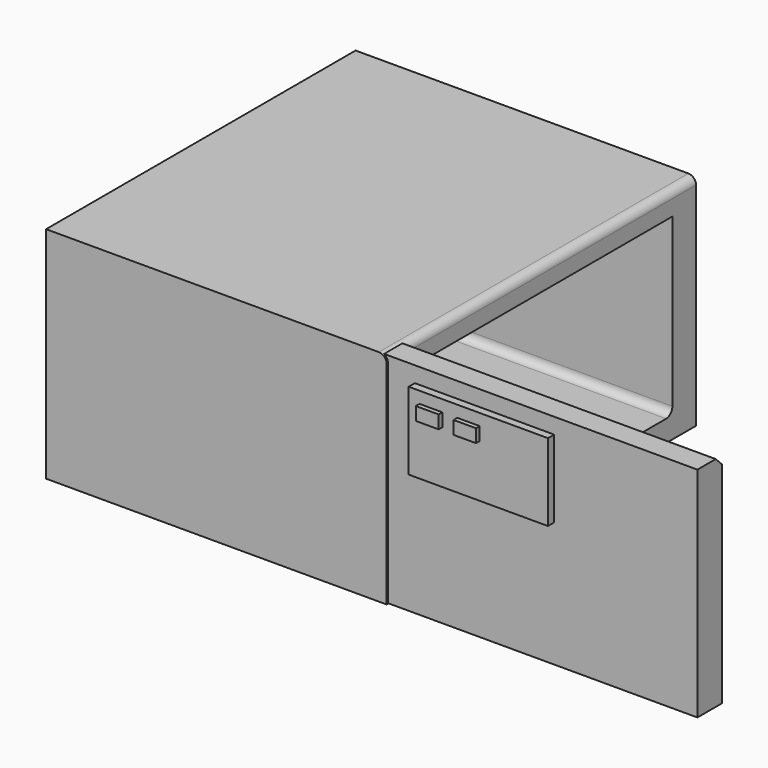
from build123d import *

# Parameters (mm, degrees)
F0_W         = 220
F0_H         = 141.9456327772
F1_DEPTH     = 250
F3_W         = 210.672037676
F3_H         = 112.9930540919
F4_DEPTH     = 206
F5_W         = 19.7831674727
F5_H         = 141
F6_DEPTH     = 200
F7_T4_DEPTH  = 275
F7_T10_DEPTH = 275
F7_T16_DEPTH = 275
F7_T23_DEPTH = 275
F7_T29_DEPTH = 275
F8_SIZE      = 5
F9_T1_DEPTH  = 218.5
F10_R        = 5
F11_R        = 5
F12_W        = 90
F12_H        = 50
F13_DEPTH    = 5
F14_W        = 14.7826219899
F14_H        = 8.5
F15_DEPTH    = 3
F16_W        = 14.5
F16_H        = 8.5
F17_DEPTH    = 3


# Not quite as in the source:
# - a fillet or chamfer that OpenCascade refuses, or shapes differently, is made with other operations: its cross-section is extruded or revolved along the edge and cut away or added


with BuildPart() as f1:
    # F0 (on Front) → F1 (new body)
    with BuildSketch(Plane.XZ):
        Rectangle(F0_W, F0_H)
    extrude(amount=F1_DEPTH)

    # F3 (on face) → F4 (cut)
    with BuildSketch(Plane.YZ.offset(110)):
        with Locations((-124.4797622785, -0.6201006472)):
            Rectangle(F3_W, F3_H)
    extrude(amount=-F4_DEPTH, mode=Mode.SUBTRACT)

    # F5 (on face) → F6 (join)
    with BuildSketch(Plane.YZ.offset(110)):
        with Locations((-239.0063405037, -0.1803636551)):
            Rectangle(F5_W, F5_H)
    extrude(amount=F6_DEPTH)

    # F7: fillet of radius 5 on 1 edges, made by hand


with BuildPart() as f7_tool2:
    # F7_s3 → F7_t4 (new body)
    with BuildSketch(Plane.XZ.offset(-12.5)):
        with BuildLine():
            ThreePointArc((105, 70.9728163886), (108.5355339059, 69.5083502945), (110, 65.9728163886))
            Line((110, 65.9728163886), (110, 70.9728163886))
            Line((110, 70.9728163886), (105, 70.9728163886))
        make_face()
    extrude(amount=F7_T4_DEPTH)

    split(bisect_by=Plane.XY.offset(70.3196363449), keep=Keep.TOP)

    split(bisect_by=Plane.XZ.offset(229.1147567674), keep=Keep.BOTTOM)


with BuildPart() as f1_1:
    add(f1.part)

    # F7_t1: cut F7_tool2
    add(f7_tool2.part, mode=Mode.SUBTRACT)


with BuildPart() as f7_tool8:
    # F7_s9 → F7_t10 (new body)
    with BuildSketch(Plane.XZ.offset(-12.5)):
        with BuildLine():
            ThreePointArc((105, 70.9728163886), (108.5355339059, 69.5083502945), (110, 65.9728163886))
            Line((110, 65.9728163886), (110, 70.9728163886))
            Line((110, 70.9728163886), (105, 70.9728163886))
        make_face()
    extrude(amount=F7_T10_DEPTH)

    split(bisect_by=Plane.XY.offset(70.3196363449), keep=Keep.BOTTOM)

    split(bisect_by=Plane.XZ.offset(229.1147567674), keep=Keep.BOTTOM)


with BuildPart() as f1_2:
    add(f1_1.part)

    # F7_t7: cut F7_tool8
    add(f7_tool8.part, mode=Mode.SUBTRACT)


with BuildPart() as f7_tool14:
    # F7_s15 → F7_t16 (new body)
    with BuildSketch(Plane.XZ.offset(-12.5)):
        with BuildLine():
            ThreePointArc((105, 70.9728163886), (108.5355339059, 69.5083502945), (110, 65.9728163886))
            Line((110, 65.9728163886), (110, 70.9728163886))
            Line((110, 70.9728163886), (105, 70.9728163886))
        make_face()
    extrude(amount=F7_T16_DEPTH)

    split(bisect_by=Plane.XZ.offset(248.89792424), keep=Keep.BOTTOM)

    split(bisect_by=Plane.XY.offset(70.3196363449), keep=Keep.TOP)

    split(bisect_by=Plane.XZ.offset(229.1147567674), keep=Keep.TOP)


with BuildPart() as f1_3:
    add(f1_2.part)

    # F7_t13: cut F7_tool14
    add(f7_tool14.part, mode=Mode.SUBTRACT)


with BuildPart() as f7_tool21:
    # F7_s22 → F7_t23 (new body)
    with BuildSketch(Plane.XZ.offset(-12.5)):
        with BuildLine():
            ThreePointArc((105, 70.9728163886), (108.5355339059, 69.5083502945), (110, 65.9728163886))
            Line((110, 65.9728163886), (110, 70.9728163886))
            Line((110, 70.9728163886), (105, 70.9728163886))
        make_face()
    extrude(amount=F7_T23_DEPTH)

    split(bisect_by=Plane.XZ.offset(248.89792424), keep=Keep.TOP)

    split(bisect_by=Plane.XY.offset(70.3196363449), keep=Keep.TOP)


with BuildPart() as f1_4:
    add(f1_3.part)

    # F7_t20: cut F7_tool21
    add(f7_tool21.part, mode=Mode.SUBTRACT)


with BuildPart() as f7_tool27:
    # F7_s28 → F7_t29 (new body)
    with BuildSketch(Plane.XZ.offset(-12.5)):
        with BuildLine():
            ThreePointArc((105, 70.9728163886), (108.5355339059, 69.5083502945), (110, 65.9728163886))
            Line((110, 65.9728163886), (110, 70.9728163886))
            Line((110, 70.9728163886), (105, 70.9728163886))
        make_face()
    extrude(amount=F7_T29_DEPTH)

    split(bisect_by=Plane.XZ.offset(248.89792424), keep=Keep.TOP)

    split(bisect_by=Plane.XY.offset(70.3196363449), keep=Keep.BOTTOM)


with BuildPart() as f1_5:
    add(f1_4.part)

    # F7_t26: cut F7_tool27
    add(f7_tool27.part, mode=Mode.SUBTRACT)

    # F8
    f8_edges = [f1_5.edges().sort_by_distance(p)[0] for p in [
        (208.735431, -229.114757, 70.319636),
    ]]
    chamfer(f8_edges, length=F8_SIZE)

    # F9: fillet of radius 5 on 1 edges, made by hand

    # F9_s2 → F9_t1 (join)
    with BuildSketch(Plane.YZ.offset(-108.5)):
        with BuildLine():
            ThreePointArc((-224.8157811165, -57.1166276932), (-228.3513150224, -55.6521615991), (-229.8157811165, -52.1166276932))
            Line((-229.8157811165, -52.1166276932), (-229.8157811165, -57.1166276932))
            Line((-229.8157811165, -57.1166276932), (-224.8157811165, -57.1166276932))
        make_face()
    extrude(amount=F9_T1_DEPTH)

    # F10
    f10_edges = [f1_5.edges().sort_by_distance(p)[0] for p in [
        (-96, -121.979762, -57.116628),
    ]]
    fillet(f10_edges, radius=F10_R)

    # F11
    f11_edges = [f1_5.edges().sort_by_distance(p)[0] for p in [
        (9.5, -19.143743, -57.116628),
    ]]
    fillet(f11_edges, radius=F11_R)

    # F12 (on face) → F13 (join)
    with BuildSketch(Plane.XZ.offset(248.89792424)):
        with Locations((172.4283844233, 35.1449831093)):
            Rectangle(F12_W, F12_H)
    extrude(amount=F13_DEPTH)

    # F14 (on face) → F15 (join)
    with BuildSketch(Plane.XZ.offset(253.89792424)):
        with Locations((141.7928859591, 48.4116636217)):
            Rectangle(F14_W, F14_H)
    extrude(amount=F15_DEPTH)

    # F16 (on face) → F17 (join)
    with BuildSketch(Plane.XZ.offset(253.89792424)):
        with Locations((166.0626122952, 48.4116636217)):
            Rectangle(F16_W, F16_H)
    extrude(amount=F17_DEPTH)


solid = f1_5.part
